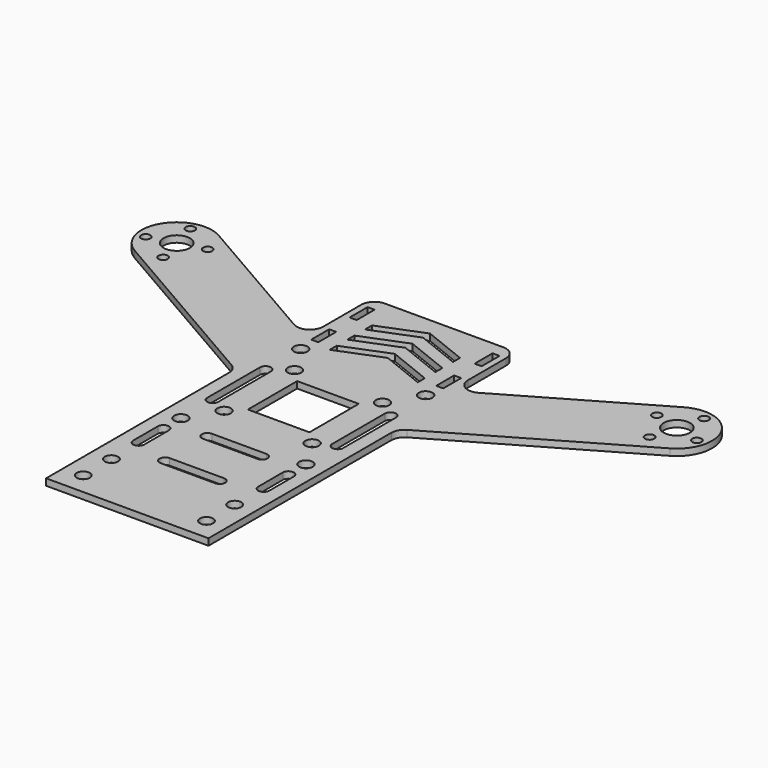
from build123d import *

# Parameters (mm, degrees)
F0_R     = 1.55
F0_W     = 1.6
F0_H     = 5.1
F0_W_2   = 14
F0_H_2   = 14
F0_R_2   = 1.05
F0_R_3   = 3
F1_DEPTH = 1.5
F2_R     = 3
F3_R     = 1.5
F4_DEPTH = 1.501


with BuildPart() as f1:
    # F0 (on Top) → F1 (new body)
    with BuildSketch(Plane.XY):
        Polygon((18.45, -32), (16.45, -32), (-16.45, -32), (-18.45, -32), (-18.45, -58), (18.45, -58), align=None)
        Polygon((-16.45, -32), (16.45, -32), (16.45, -5.4752086141), (16.45, 13), (16.45, 32), (-16.45, 32), (-16.45, 13), (-16.45, -5.4752086141), align=None)
        with Locations((-14.2, -25)):
            Circle(F0_R, mode=Mode.SUBTRACT)
        with Locations((-10, -18)):
            Circle(F0_R, mode=Mode.SUBTRACT)
        with Locations((14.2, -25)):
            Circle(F0_R, mode=Mode.SUBTRACT)
        with Locations((10, -18)):
            Circle(F0_R, mode=Mode.SUBTRACT)
        with Locations((-10, 2)):
            Circle(F0_R, mode=Mode.SUBTRACT)
        with Locations((-14.2, 9)):
            Circle(F0_R, mode=Mode.SUBTRACT)
        with Locations((-14.2, 15.55)):
            Rectangle(F0_W, F0_H, mode=Mode.SUBTRACT)
        with Locations((-14.2, 26.45)):
            Rectangle(F0_W, F0_H, mode=Mode.SUBTRACT)
        with Locations((0, -8)):
            Rectangle(F0_W_2, F0_H_2, mode=Mode.SUBTRACT)
        with Locations((10, 2)):
            Circle(F0_R, mode=Mode.SUBTRACT)
        with Locations((14.2, 9)):
            Circle(F0_R, mode=Mode.SUBTRACT)
        Polygon((-10, 14), (0, 18), (10, 14), (10, 12), (0, 16), (-10, 12), align=None, mode=Mode.SUBTRACT)
        with Locations((14.2, 15.55)):
            Rectangle(F0_W, F0_H, mode=Mode.SUBTRACT)
        Polygon((-10, 19), (0, 23), (10, 19), (10, 17), (0, 21), (-10, 17), align=None, mode=Mode.SUBTRACT)
        Polygon((-10, 24), (0, 28), (10, 24), (10, 22), (0, 26), (-10, 22), align=None, mode=Mode.SUBTRACT)
        with Locations((14.2, 26.45)):
            Rectangle(F0_W, F0_H, mode=Mode.SUBTRACT)
        Polygon((16.45, -5.4752086141), (16.45, -32), (18.45, -32), (18.45, -4.3205080757), align=None)
        Polygon((-18.45, -32), (-16.45, -32), (-16.45, -5.4752086141), (-18.45, -4.3205080757), align=None)
        with BuildLine():
            Line((16.45, 13), (16.45, -5.4752086141))
            Line((16.45, -5.4752086141), (18.45, -4.3205080757))
            Line((18.45, -4.3205080757), (60.8230669589, 20.1435935394))
            ThreePointArc((60.8230669589, 20.1435935394), (63.7512701892, 31.0717967697), (52.8230669589, 34))
            Line((52.8230669589, 34), (16.45, 13))
        make_face()
        with Locations((55.2701526883, 21.276241812)):
            Circle(F0_R_2, mode=Mode.SUBTRACT)
        with Locations((51.0275120012, 28.6247110403)):
            Circle(F0_R_2, mode=Mode.SUBTRACT)
        with Locations((62.6186219167, 25.5188824991)):
            Circle(F0_R_2, mode=Mode.SUBTRACT)
        with Locations((56.8230669589, 27.0717967697)):
            Circle(F0_R_3, mode=Mode.SUBTRACT)
        with Locations((58.3759812296, 32.8673517275)):
            Circle(F0_R_2, mode=Mode.SUBTRACT)
        with BuildLine():
            Line((-18.45, -4.3205080757), (-16.45, -5.4752086141))
            Line((-16.45, -5.4752086141), (-16.45, 13))
            Line((-16.45, 13), (-52.8230669589, 34))
            ThreePointArc((-52.8230669589, 34), (-63.7512701892, 31.0717967697), (-60.8230669589, 20.1435935394))
            Line((-60.8230669589, 20.1435935394), (-18.45, -4.3205080757))
        make_face()
        with Locations((-55.2701526883, 21.276241812)):
            Circle(F0_R_2, mode=Mode.SUBTRACT)
        with Locations((-62.6186219167, 25.5188824991)):
            Circle(F0_R_2, mode=Mode.SUBTRACT)
        with Locations((-56.8230669589, 27.0717967697)):
            Circle(F0_R_3, mode=Mode.SUBTRACT)
        with Locations((-51.0275120012, 28.6247110403)):
            Circle(F0_R_2, mode=Mode.SUBTRACT)
        with Locations((-58.3759812296, 32.8673517275)):
            Circle(F0_R_2, mode=Mode.SUBTRACT)
    extrude(amount=F1_DEPTH)

    # F2
    f2_edges = [f1.edges().sort_by_distance(p)[0] for p in [
        (-16.45, 13, 0.75),
        (16.45, 13, 0.75),
        (18.45, -4.320508, 0.75),
        (-18.45, -4.320508, 0.75),
        (16.45, 32, 0.75),
        (-16.45, 32, 0.75),
    ]]
    fillet(f2_edges, radius=F2_R)

    # F3 (on face) → F4 (cut, through all)
    with BuildSketch(Plane.XY.offset(1.5)):
        with BuildLine():
            ThreePointArc((-12.95, -1), (-14.2, 0.25), (-15.45, -1))
            Line((-15.45, -1), (-15.45, -16))
            ThreePointArc((-15.45, -16), (-14.2, -17.25), (-12.95, -16))
            Line((-12.95, -16), (-12.95, -1))
        make_face()
        with BuildLine():
            ThreePointArc((15.45, -1), (14.2, 0.25), (12.95, -1))
            Line((12.95, -1), (12.95, -16))
            ThreePointArc((12.95, -16), (14.2, -17.25), (15.45, -16))
            Line((15.45, -16), (15.45, -1))
        make_face()
        with BuildLine():
            ThreePointArc((-12.95, -30), (-14.2, -28.75), (-15.45, -30))
            Line((-15.45, -30), (-15.45, -37))
            ThreePointArc((-15.45, -37), (-14.2, -38.25), (-12.95, -37))
            Line((-12.95, -37), (-12.95, -30))
        make_face()
        with BuildLine():
            ThreePointArc((15.45, -30), (14.2, -28.75), (12.95, -30))
            Line((12.95, -30), (12.95, -37))
            ThreePointArc((12.95, -37), (14.2, -38.25), (15.45, -37))
            Line((15.45, -37), (15.45, -30))
        make_face()
        with Locations((-14, -45)):
            Circle(F3_R)
        with Locations((-14, -53)):
            Circle(F3_R)
        with Locations((14, -45)):
            Circle(F3_R)
        with Locations((14, -53)):
            Circle(F3_R)
        with BuildLine():
            ThreePointArc((-6.2, -26.25), (-7.45, -27.5), (-6.2, -28.75))
            Line((-6.2, -28.75), (6.2, -28.75))
            ThreePointArc((6.2, -28.75), (7.45, -27.5), (6.2, -26.25))
            Line((6.2, -26.25), (-6.2, -26.25))
        make_face()
        with BuildLine():
            ThreePointArc((-6.2, -38.25), (-7.45, -39.5), (-6.2, -40.75))
            Line((-6.2, -40.75), (6.2, -40.75))
            ThreePointArc((6.2, -40.75), (7.45, -39.5), (6.2, -38.25))
            Line((6.2, -38.25), (-6.2, -38.25))
        make_face()
    extrude(amount=-F4_DEPTH, mode=Mode.SUBTRACT)


solid = f1.part
